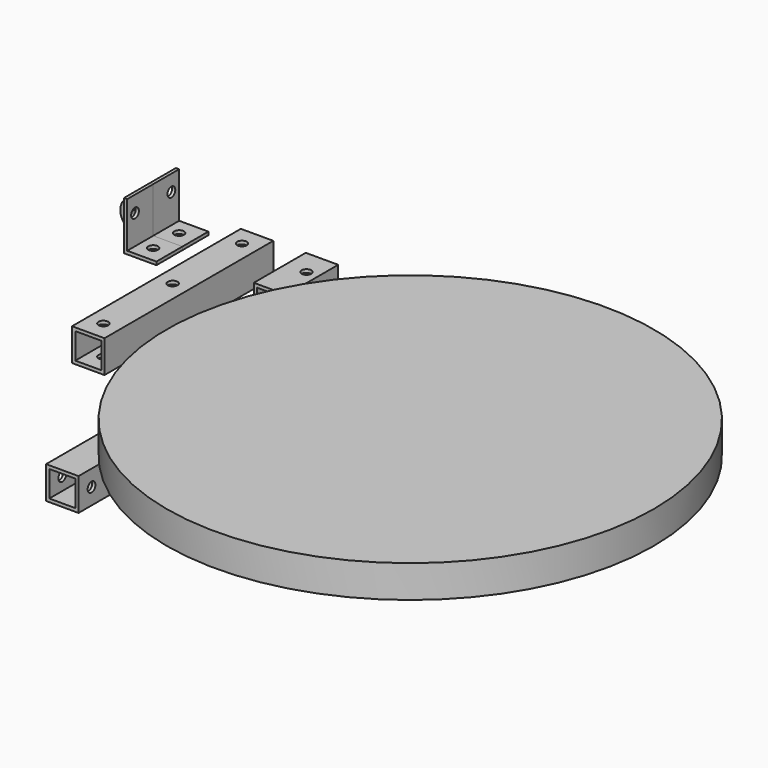
from build123d import *

# Parameters (mm, degrees)
F0_W      = 20
F0_H      = 20
F0_W_2    = 16
F0_H_2    = 16
F1_DEPTH  = 220
F2_R      = 3
F3_DEPTH  = 20
F4_R      = 3
F5_DEPTH  = 2
F6_R      = 6
F7_R      = 3
F8_DEPTH  = 2
F9_R      = 5
F10_DEPTH = 2
F11_W     = 15
F11_H     = 62
F11_R     = 3
F12_DEPTH = 5
F14_DEPTH = 50
F15_R     = 3
F16_DEPTH = 2
F17_R     = 3
F18_DEPTH = 20
F19_R     = 6
F20_R     = 1.99999
F21_R     = 3
F22_DEPTH = 20
F23_R     = 2
F23_R_2   = 3
F24_DEPTH = 2
F25_W     = 20
F25_H     = 20
F25_W_2   = 16
F25_H_2   = 16
F26_DEPTH = 120
F27_R     = 3
F28_DEPTH = 2
F30_DEPTH = 20
F31_R     = 1.99999
F32_R     = 150
F33_DEPTH = 20
F34_W     = 20
F34_H     = 20
F34_W_2   = 16
F34_H_2   = 16
F35_DEPTH = 250
F36_R     = 3
F37_DEPTH = 25.001
F38_R     = 3
F39_DEPTH = 286.397509233
F40_W     = 20
F40_H     = 20
F40_W_2   = 16
F40_H_2   = 16
F41_DEPTH = 40
F42_R     = 3
F43_DEPTH = 326.397509233
F44_W     = 20
F44_H     = 20
F44_W_2   = 16
F44_H_2   = 16
F45_DEPTH = 130
F46_R     = 3
F47_DEPTH = 25.001
F48_R     = 3
F49_DEPTH = 25.001
F51_DEPTH = 20
F52_R     = 3
F53_DEPTH = 2
F54_R     = 3
F55_DEPTH = 2
F56_R     = 9.5
F56_R_2   = 3
F57_DEPTH = 6
F59_DEPTH = 20
F60_R     = 3
F61_DEPTH = 2
F62_R     = 3
F63_DEPTH = 2


# Not quite as in the source:
# - a fillet or chamfer is up to 0.001 mm smaller than in the source, because OpenCascade refuses the exact size


with BuildPart() as f1:
    # F0 (on Front) → F1 (new body)
    with BuildSketch(Plane.XZ):
        Rectangle(F0_W, F0_H)
        Rectangle(F0_W_2, F0_H_2, mode=Mode.SUBTRACT)
    extrude(amount=F1_DEPTH)

    # F2 (on face) → F3 (cut, through all)
    with BuildSketch(Plane.XY.offset(10)):
        with Locations((0, -30)):
            Circle(F2_R)
        with Locations((0, -70)):
            Circle(F2_R)
        with Locations((0, -210)):
            Circle(F2_R)
    extrude(amount=-F3_DEPTH, mode=Mode.SUBTRACT)

    # F7 (on face) → F8 (cut, through all)
    with BuildSketch(Plane(origin=(0, 0, -10), x_dir=(1, 0, 0), z_dir=(0, 0, -1))):
        with Locations((0, 10)):
            Circle(F7_R)
    extrude(amount=-F8_DEPTH, mode=Mode.SUBTRACT)

    # F9 (on face) → F10 (cut, through all)
    with BuildSketch(Plane.XY.offset(10)):
        with Locations((0, -10)):
            Circle(F9_R)
    extrude(amount=-F10_DEPTH, mode=Mode.SUBTRACT)

    # F20 (radius 2 in the source; OpenCascade refuses exactly that, so slightly less here)
    f20_edges = [f1.edges().sort_by_distance(p)[0] for p in [
        (10, -220, 0),
        (-10, -220, 0),
        (10, 0, 0),
        (-10, 0, 0),
    ]]
    fillet(f20_edges, radius=F20_R)

    # F21 (on face) → F22 (cut, through all)
    with BuildSketch(Plane.YZ.offset(10)):
        with Locations((-140, 0)):
            Circle(F21_R)
    extrude(amount=-F22_DEPTH, mode=Mode.SUBTRACT)


with BuildPart() as f5:
    # F4 (on face) → F5 (new body)
    with BuildSketch(Plane.XY.offset(10)):
        Polygon((-8.6602540378, -15), (-8.6602540378, -85), (51.9615242271, -50), align=None)
        with Locations((0, -70)):
            Circle(F4_R, mode=Mode.SUBTRACT)
        with Locations((0, -30)):
            Circle(F4_R, mode=Mode.SUBTRACT)
        with Locations((34.6410161514, -50)):
            Circle(F4_R, mode=Mode.SUBTRACT)
    extrude(amount=F5_DEPTH)

    # F6
    f6_edges = [f5.edges().sort_by_distance(p)[0] for p in [
        (-8.660254, -85, 11),
        (-8.660254, -15, 11),
        (51.961524, -50, 11),
    ]]
    fillet(f6_edges, radius=F6_R)


with BuildPart() as f12:
    # F11 (on face) → F12 (new body)
    with BuildSketch(Plane(origin=(0, 0, -10), x_dir=(1, 0, 0), z_dir=(0, 0, -1))):
        with Locations((0, 7)):
            Rectangle(F11_W, F11_H)
        with Locations((0, -16)):
            Circle(F11_R, mode=Mode.SUBTRACT)
        with Locations((0, 10)):
            Circle(F11_R, mode=Mode.SUBTRACT)
        with Locations((0, 30)):
            Circle(F11_R, mode=Mode.SUBTRACT)
    extrude(amount=F12_DEPTH)

    # F19
    f19_edges = [f12.edges().sort_by_distance(p)[0] for p in [
        (7.5, -38, -12.5),
        (-7.5, -38, -12.5),
        (-7.5, 24, -12.5),
        (7.5, 24, -12.5),
    ]]
    fillet(f19_edges, radius=F19_R)


with BuildPart() as f14:
    # F13 (on Front) → F14 (new body)
    with BuildSketch(Plane.XZ):
        Polygon((60, 8), (60, 10), (40, 10), (40, -10), (60, -10), (60, -8), (42, -8), (42, 8), align=None)
    extrude(amount=F14_DEPTH)

    # F15 (on face) → F16 (cut, through all)
    with BuildSketch(Plane(origin=(0, 0, -10), x_dir=(1, 0, 0), z_dir=(0, 0, -1))):
        with Locations((52, 25)):
            Circle(F15_R)
        with Locations((52, 8)):
            Circle(F15_R)
    extrude(amount=-F16_DEPTH, mode=Mode.SUBTRACT)

    # F17 (on face) → F18 (cut, through all)
    with BuildSketch(Plane.XY.offset(10)):
        with Locations((51.9999999998, -42)):
            Circle(F17_R)
    extrude(amount=-F18_DEPTH, mode=Mode.SUBTRACT)


with BuildPart() as f24:
    # F23 (on face) → F24 (new body)
    with BuildSketch(Plane.XY.offset(12)):
        with BuildLine():
            ThreePointArc((-64.2511678583, -110), (-64.2511678583, -114), (-60.7870662432, -116))
            Line((-60.7870662432, -116), (15.0111069989, -116))
            ThreePointArc((15.0111069989, -116), (18.4752086141, -114), (18.4752086141, -110))
            Line((18.4752086141, -110), (-19.423878007, -44.3568564119))
            ThreePointArc((-19.423878007, -44.3568564119), (-22.8879796221, -42.3568564119), (-26.3520812373, -44.3568564119))
            Line((-26.3520812373, -44.3568564119), (-64.2511678583, -110))
        make_face()
        with Locations((-57.322964628, -110)):
            Circle(F23_R, mode=Mode.SUBTRACT)
        with Locations((-22.8879796221, -90.1189521373)):
            Circle(F23_R_2, mode=Mode.SUBTRACT)
        with Locations((11.5470053838, -110)):
            Circle(F23_R, mode=Mode.SUBTRACT)
        with Locations((-22.8879796221, -50.3568564119)):
            Circle(F23_R, mode=Mode.SUBTRACT)
    extrude(amount=F24_DEPTH)


with BuildPart() as f26:
    # F25 (on Front) → F26 (new body)
    with BuildSketch(Plane.XZ):
        with Locations((-22.8879796221, 0)):
            Rectangle(F25_W, F25_H)
        with Locations((-22.8879796221, 0)):
            Rectangle(F25_W_2, F25_H_2, mode=Mode.SUBTRACT)
    extrude(amount=F26_DEPTH)

    # F27 (on face) → F28 (cut, through all)
    with BuildSketch(Plane.XY.offset(10)):
        with Locations((-22.8879796221, -10)):
            Circle(F27_R)
        with Locations((-22.8879796221, -110)):
            Circle(F27_R)
    extrude(amount=-F28_DEPTH, mode=Mode.SUBTRACT)

    # F29 (on face) → F30 (cut, through all)
    with BuildSketch(Plane(origin=(-32.8879796221, 0, 0), x_dir=(0, -1, 0), z_dir=(-1, 0, 0))):
        with BuildLine():
            ThreePointArc((60, -3), (62.1213203436, -2.1213203436), (63, 0))
            ThreePointArc((63, 0), (57.8786796564, 2.1213203436), (60, -3))
        make_face()
    extrude(amount=-F30_DEPTH, mode=Mode.SUBTRACT)

    # F31 (radius 2 in the source; OpenCascade refuses exactly that, so slightly less here)
    f31_edges = [f26.edges().sort_by_distance(p)[0] for p in [
        (-32.88798, -120, 0),
        (-12.88798, -120, 0),
        (-32.88798, 0, 0),
        (-12.88798, 0, 0),
    ]]
    fillet(f31_edges, radius=F31_R)


with BuildPart() as f33:
    # F32 (on face) → F33 (new body)
    with BuildSketch(Plane.XY.offset(14)):
        with Locations((63.5085296109, -140)):
            Circle(F32_R)
    extrude(amount=F33_DEPTH)


with BuildPart() as f35:
    # F34 (on Front) → F35 (new body)
    with BuildSketch(Plane.XZ):
        with Locations((-62.8879796221, 0)):
            Rectangle(F34_W, F34_H)
        with Locations((-62.8879796221, 0)):
            Rectangle(F34_W_2, F34_H_2, mode=Mode.SUBTRACT)
    extrude(amount=F35_DEPTH)

    # F36 (on face) → F37 (cut, through all)
    with BuildSketch(Plane.XY.offset(10)):
        with Locations((-62.8879796221, -105)):
            Circle(F36_R)
        with Locations((-62.8879796221, -145)):
            Circle(F36_R)
    extrude(amount=-F37_DEPTH, mode=Mode.SUBTRACT)

    # F38 (on face) → F39 (cut, through all)
    with BuildSketch(Plane(origin=(-72.8879796221, 0, 0), x_dir=(0, -1, 0), z_dir=(-1, 0, 0))):
        with Locations((10, 0)):
            Circle(F38_R)
        with Locations((30, 0)):
            Circle(F38_R)
        with Locations((220, 0)):
            Circle(F38_R)
        with Locations((240, 0)):
            Circle(F38_R)
    extrude(amount=-F39_DEPTH, mode=Mode.SUBTRACT)


with BuildPart() as f41:
    # F40 (on Front) → F41 (new body)
    with BuildSketch(Plane.XZ):
        with Locations((-102.8879796221, 0)):
            Rectangle(F40_W, F40_H)
        with Locations((-102.8879796221, 0)):
            Rectangle(F40_W_2, F40_H_2, mode=Mode.SUBTRACT)
    extrude(amount=F41_DEPTH)

    # F42 (on face) → F43 (cut, through all)
    with BuildSketch(Plane(origin=(-112.8879796221, 0, 0), x_dir=(0, -1, 0), z_dir=(-1, 0, 0))):
        with Locations((10, 0)):
            Circle(F42_R)
        with Locations((30, 0)):
            Circle(F42_R)
    extrude(amount=-F43_DEPTH, mode=Mode.SUBTRACT)

    # F48 (on face) → F49 (cut, through all)
    with BuildSketch(Plane.XY.offset(10)):
        with Locations((-100.0949796221, -15.417)):
            Circle(F48_R)
    extrude(amount=-F49_DEPTH, mode=Mode.SUBTRACT)


with BuildPart() as f45:
    # F44 (on Front) → F45 (new body)
    with BuildSketch(Plane.XZ):
        with Locations((-142.8879796221, 0)):
            Rectangle(F44_W, F44_H)
        with Locations((-142.8879796221, 0)):
            Rectangle(F44_W_2, F44_H_2, mode=Mode.SUBTRACT)
    extrude(amount=F45_DEPTH)

    # F46 (on face) → F47 (cut, through all)
    with BuildSketch(Plane.XY.offset(10)):
        with Locations((-142.8879796221, -65)):
            Circle(F46_R)
        with Locations((-142.8879796221, -11.632)):
            Circle(F46_R)
        with Locations((-142.8879796221, -118.368)):
            Circle(F46_R)
    extrude(amount=-F47_DEPTH, mode=Mode.SUBTRACT)


with BuildPart() as f51:
    # F50 (on Front) → F51 (new body)
    with BuildSketch(Plane.XZ):
        Polygon((-192.8879796221, 0), (-172.8879796221, 0), (-172.8879796221, 2), (-190.8879796221, 2), (-190.8879796221, 30), (-192.8879796221, 30), align=None)
    extrude(amount=F51_DEPTH)

    # F52 (on face) → F53 (cut, through all)
    with BuildSketch(Plane(origin=(0, 0, 0), x_dir=(1, 0, 0), z_dir=(0, 0, -1))):
        with Locations((-182.8879796221, 10)):
            Circle(F52_R)
    extrude(amount=-F53_DEPTH, mode=Mode.SUBTRACT)

    # F54 (on face) → F55 (cut, through all)
    with BuildSketch(Plane(origin=(-192.8879796221, 0, 0), x_dir=(0, -1, 0), z_dir=(-1, 0, 0))):
        with Locations((6, 20)):
            Circle(F54_R)
    extrude(amount=-F55_DEPTH, mode=Mode.SUBTRACT)


with BuildPart() as f57:
    # F56 (on Front) → F57 (new body)
    with BuildSketch(Plane.XZ):
        with Locations((-212.8879796221, 0)):
            Circle(F56_R)
        with Locations((-212.8879796221, 0)):
            Circle(F56_R_2, mode=Mode.SUBTRACT)
    extrude(amount=F57_DEPTH)


with BuildPart() as f59:
    # F58 (on face) → F59 (new body)
    with BuildSketch(Plane.XZ.offset(20)):
        Polygon((-190.8879796221, 30), (-192.8879796221, 30), (-192.8879796221, 0), (-172.8879796221, 0), (-172.8879796221, 2), (-190.8879796221, 2), align=None)
    extrude(amount=F59_DEPTH)

    # F60 (on face) → F61 (cut, through all)
    with BuildSketch(Plane(origin=(0, 0, 0), x_dir=(1, 0, 0), z_dir=(0, 0, -1))):
        with Locations((-182.8879796221, 30)):
            Circle(F60_R)
    extrude(amount=-F61_DEPTH, mode=Mode.SUBTRACT)

    # F62 (on face) → F63 (cut, through all)
    with BuildSketch(Plane(origin=(-192.8879796221, 0, 0), x_dir=(0, -1, 0), z_dir=(-1, 0, 0))):
        with Locations((34, 20)):
            Circle(F62_R)
    extrude(amount=-F63_DEPTH, mode=Mode.SUBTRACT)


solid = Compound([f1.part, f5.part, f12.part, f14.part, f24.part, f26.part, f33.part, f35.part, f41.part, f45.part, f51.part, f57.part, f59.part])
